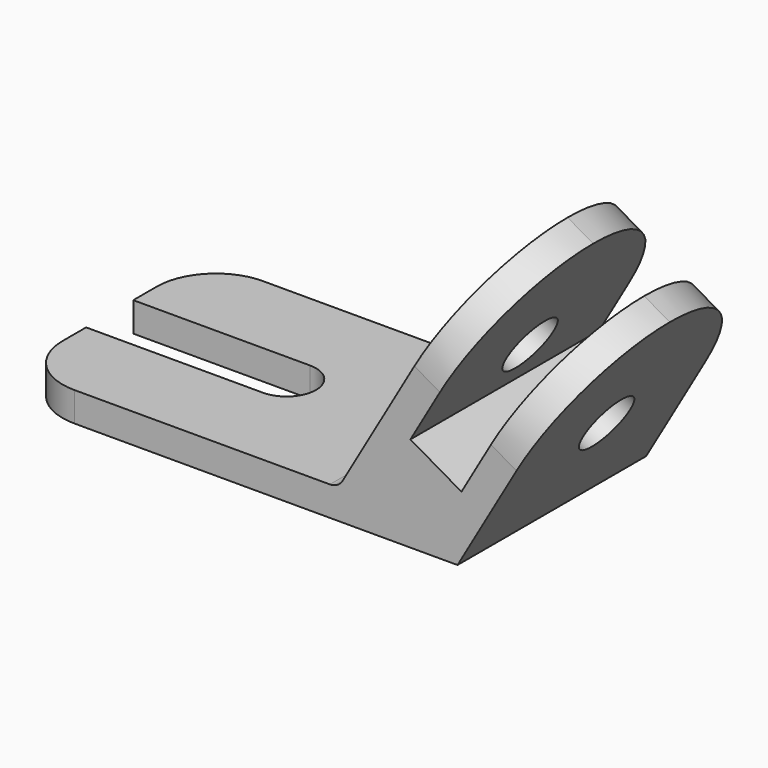
from build123d import *

# Parameters (mm, degrees)
F1_DEPTH = 40
F2_R     = 39.99999
F3_R     = 20
F5_D     = 20
F6_R     = 5
F8_DEPTH = 10.001


# Not quite as in the source:
# - a fillet or chamfer is up to 0.001 mm smaller than in the source, because OpenCascade refuses the exact size


with BuildPart() as f1:
    # F0 (on Front) → F1 (new body, symmetric)
    with BuildSketch(Plane.XZ):
        Polygon((0, 10), (0, 0), (150, 0), (190, 69.2820323028), (181.3397459622, 74.2820323028), (151.3397459622, 22.3205080757), (134.0192378865, 32.3205080757), (164.0192378865, 84.2820323028), (155.3589838486, 89.2820323028), (109.5854811567, 10), align=None)
    extrude(amount=F1_DEPTH, both=True)

    # F2 (radius 40 in the source; OpenCascade refuses exactly that, so slightly less here)
    f2_edges = [f1.edges().sort_by_distance(p)[0] for p in [
        (159.689111, -40, 86.782032),
        (159.689111, 40, 86.782032),
        (185.669873, 40, 71.782032),
        (185.669873, -40, 71.782032),
    ]]
    fillet(f2_edges, radius=F2_R)

    # F3
    f3_edges = [f1.edges().sort_by_distance(p)[0] for p in [
        (0, -40, 5),
        (0, 40, 5),
    ]]
    fillet(f3_edges, radius=F3_R)

    # F5 (through all)
    with Locations(Plane(origin=(77.8589838486, 0, -44.9519052838), x_dir=(0, -1, 0), z_dir=(-0.8660254038, 0, 0.5))):
        with Locations((0, 112.1529946162)):
            Hole(F5_D / 2)

    # F6
    f6_edges = [f1.edges().sort_by_distance(p)[0] for p in [
        (109.585481, 0, 10),
    ]]
    fillet(f6_edges, radius=F6_R)

    # F7 (on face) → F8 (cut, through all)
    with BuildSketch(Plane.XY.offset(10)):
        with BuildLine():
            Line((0, 0), (0, -10))
            Line((0, -10), (60, -10))
            ThreePointArc((60, -10), (70, 0), (60, 10))
            Line((60, 10), (0, 10))
            Line((0, 10), (0, 0))
        make_face()
    extrude(amount=-F8_DEPTH, mode=Mode.SUBTRACT)


solid = f1.part
